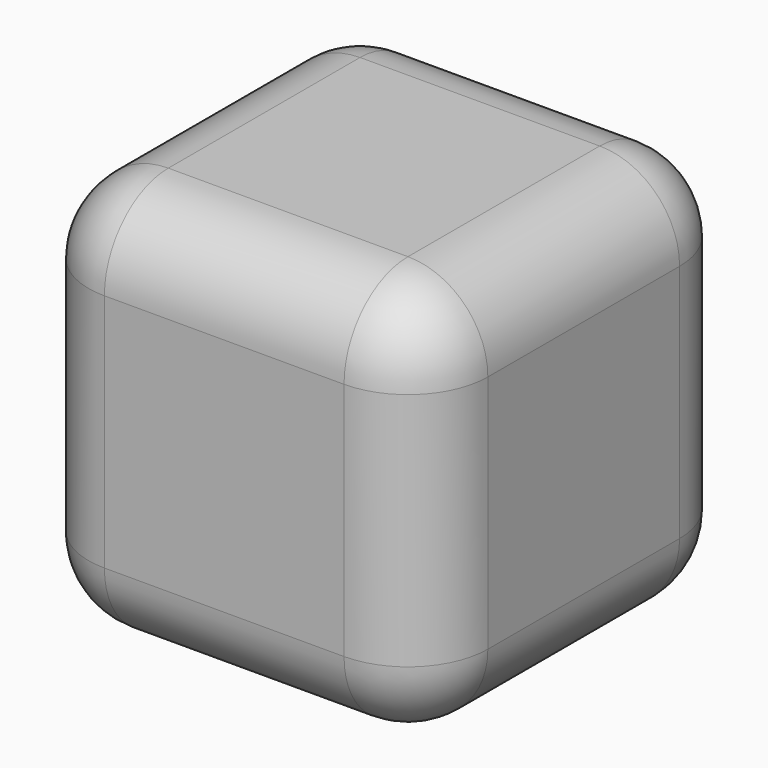
from build123d import *

# Parameters (mm, degrees)
F0_W     = 25
F0_H     = 25
F1_DEPTH = 25
F2_R     = 5
F3_T     = -3


# Not quite as in the source:
# - a shell that OpenCascade refuses in one call is made with other operations: the cavity is built on its own and cut out


with BuildPart() as f1:
    # F0 (on Top) → F1 (new body)
    with BuildSketch(Plane.XY):
        with Locations((12.5, 12.5)):
            Rectangle(F0_W, F0_H)
    extrude(amount=F1_DEPTH)

    # F2
    f2_edges = [f1.edges().sort_by_distance(p)[0] for p in [
        (12.5, 0, 0),
        (25, 0, 12.5),
        (12.5, 0, 25),
        (25, 25, 12.5),
        (25, 12.5, 0),
        (25, 12.5, 25),
        (0, 25, 12.5),
        (0, 0, 12.5),
        (0, 12.5, 0),
        (0, 12.5, 25),
        (12.5, 25, 0),
        (12.5, 25, 25),
    ]]
    fillet(f2_edges, radius=F2_R)

    # F3: a shell. OpenCascade refuses it in one call, so the cavity is built on its own and cut out:
    # the body offset inwards by the wall thickness, plus a prism from it out through each open face.
    f3_core = offset(f1.part, amount=F3_T, mode=Mode.PRIVATE)
    f3_exits = [f3_core.faces().sort_by_distance(p)[0] for p in [
        (12.5, 12.5, 3),
    ]]
    add(f3_core, mode=Mode.SUBTRACT)
    extrude(f3_exits, amount=-F3_T, mode=Mode.SUBTRACT)


solid = f1.part
